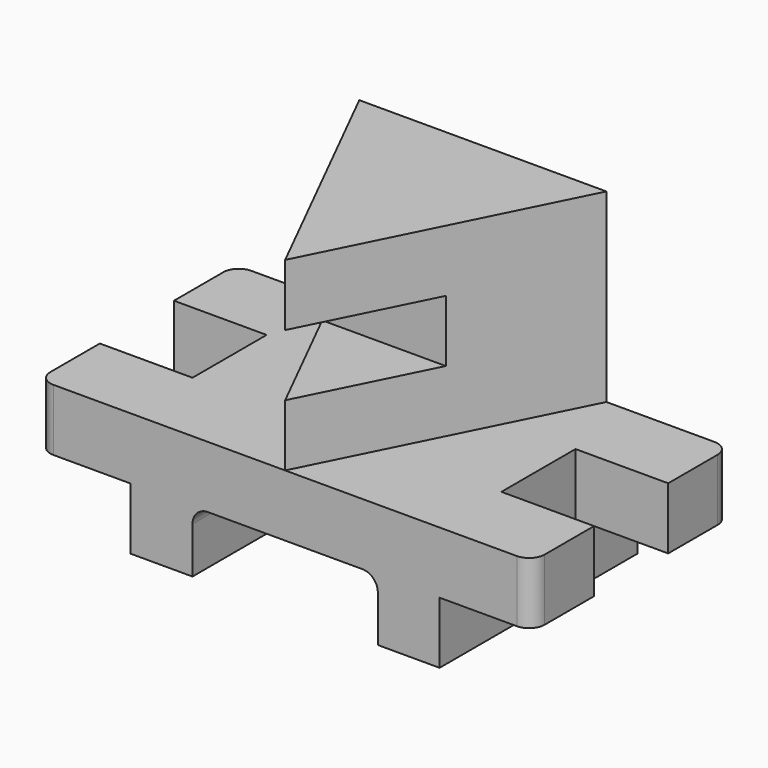
from build123d import *

# Parameters (mm, degrees)
F1_DEPTH  = 50.8
F2_R      = 6.35
F3_R      = 6.35
F4_W      = 38.1
F4_H      = 25.4
F5_DEPTH  = 38.1
F6_W      = 38.1
F6_H      = 25.4
F7_DEPTH  = 38.1
F8_W      = 101.6
F8_H      = 101.6
F9_DEPTH  = 76.2
F10_W     = 50.8
F10_H     = 25.4
F11_DEPTH = 152.401
F13_DEPTH = 76.2
F14_DEPTH = 76.2


# Not quite as in the source:
# - a feature names something its author has since deleted; it is built from what else it names


with BuildPart() as f1:
    # F0 (on Front) → F1 (new body, symmetric)
    with BuildSketch(Plane.XZ):
        Polygon((0, 25.4), (0, 0), (25.4, 0), (25.4, 25.4), (101.6, 25.4), (101.6, 0), (127, 0), (127, 25.4), (165.1, 25.4), (165.1, 50.8), (-38.1, 50.8), (-38.1, 25.4), align=None)
    extrude(amount=F1_DEPTH, both=True)

    # F2
    f2_edges = [f1.edges().sort_by_distance(p)[0] for p in [
        (165.1, -50.8, 38.1),
        (165.1, 50.8, 38.1),
        (-38.1, -50.8, 38.1),
        (-38.1, 50.8, 38.1),
    ]]
    fillet(f2_edges, radius=F2_R)

    # F3
    f3_edges = [f1.edges().sort_by_distance(p)[0] for p in [
        (25.4, 0, 25.4),
        (101.6, 0, 25.4),
    ]]
    fillet(f3_edges, radius=F3_R)

    # F4 (on face) → F5 (cut)
    with BuildSketch(Plane.YZ.offset(165.1)):
        with Locations((0, 38.1)):
            Rectangle(F4_W, F4_H)
    extrude(amount=-F5_DEPTH, mode=Mode.SUBTRACT)

    # F6 (on Right) → F7 (cut)
    with BuildSketch(Plane.YZ):
        with Locations((0, 38.1)):
            Rectangle(F6_W, F6_H)
    extrude(amount=-F7_DEPTH, mode=Mode.SUBTRACT)

    # F8 (on face) → F9 (join)
    with BuildSketch(Plane.XY.offset(50.8)):
        with Locations((63.5, 0)):
            Rectangle(F8_W, F8_H)
    extrude(amount=F9_DEPTH)

    # F10 (on face) → F11 (cut, through all)
    with BuildSketch(Plane.YZ.offset(114.3)):
        with Locations((-25.4, 88.9)):
            Rectangle(F10_W, F10_H)
    extrude(amount=-F11_DEPTH, mode=Mode.SUBTRACT)

    # F12 (on face) → F13 (cut, through all)
    with BuildSketch(Plane.XY.offset(127)):
        Polygon((12.7, -50.8), (63.5, -50.8), (12.7, 50.8), align=None)
    extrude(amount=-F13_DEPTH, mode=Mode.SUBTRACT)

    # F12 (on face) → F14 (cut, through all)
    with BuildSketch(Plane.XY.offset(127)):
        Polygon((114.3, 50.8), (63.5, -50.8), (114.3, -50.8), align=None)
    extrude(amount=-F14_DEPTH, mode=Mode.SUBTRACT)


solid = f1.part
